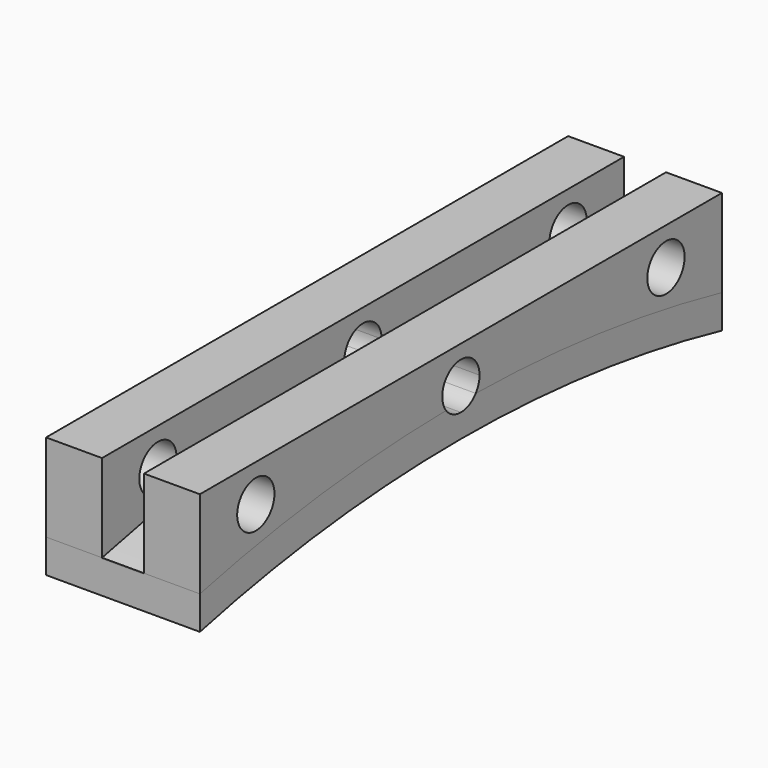
from build123d import *
from build123d import SkipClean  # not in build123d's __all__

# Parameters (mm, degrees)
F0_R     = 5
F1_DEPTH = 33
F2_W     = 9
F2_H     = 19
F3_DEPTH = 140
F5_DEPTH = 33


with BuildPart() as f1:
    # F0 (on Right) → F1 (new body)
    with BuildSketch(Plane.YZ):
        with BuildLine():
            ThreePointArc((0, 8), (35.2278299076, 5.9935116916), (70, 0))
            Line((70, 0), (70, 7.1810302798))
            ThreePointArc((70, 7.1810302798), (37.1952808389, 12.8120154562), (3.9811421818, 14.975019516))
            ThreePointArc((3.9811421818, 14.975019516), (2.2220595829, 13.5208872296), (0, 13))
            Line((0, 13), (0, 8))
        make_face()
        with BuildLine():
            ThreePointArc((3.9811421818, 14.975019516), (37.1952808389, 12.8120154562), (70, 7.1810302798))
            Line((70, 7.1810302798), (70, 26))
            Line((70, 26), (0, 26))
            Line((0, 26), (0, 23))
            ThreePointArc((0, 23), (3.5355339059, 21.5355339059), (5, 18))
            ThreePointArc((5, 18), (4.7384444129, 16.4040223856), (3.9811421818, 14.975019516))
        make_face()
        with Locations((55, 18)):
            Circle(F0_R, mode=Mode.SUBTRACT)
        with BuildLine():
            Line((-70, 26), (-70, 7.1810302798))
            ThreePointArc((-70, 7.1810302798), (-37.1952808389, 12.8120154562), (-3.9811421818, 14.975019516))
            ThreePointArc((-3.9811421818, 14.975019516), (-4.4791127704, 20.2220595829), (0, 23))
            Line((0, 23), (0, 26))
            Line((0, 26), (-70, 26))
        make_face()
        with Locations((-55, 18)):
            Circle(F0_R, mode=Mode.SUBTRACT)
        with BuildLine():
            Line((-70, 7.1810302798), (-70, 0))
            ThreePointArc((-70, 0), (-35.2278299076, 5.9935116916), (0, 8))
            Line((0, 8), (0, 13))
            ThreePointArc((0, 13), (-2.2220595829, 13.5208872296), (-3.9811421818, 14.975019516))
            ThreePointArc((-3.9811421818, 14.975019516), (-37.1952808389, 12.8120154562), (-70, 7.1810302798))
        make_face()
    extrude(amount=F1_DEPTH)

    # F2 (on face) → F3 (cut)
    with BuildSketch(Plane.XZ.offset(70)):
        with Locations((16.5, 16.5)):
            Rectangle(F2_W, F2_H)
    extrude(amount=-F3_DEPTH, mode=Mode.SUBTRACT)

    # F4 (on face) → F5 (join)
    with BuildSketch(Plane.YZ.offset(33)):
        with BuildLine():
            Line((70, 0), (70, 7.1810302798))
            ThreePointArc((70, 7.1810302798), (37.1952808389, 12.8120154562), (3.9811421818, 14.975019516))
            ThreePointArc((3.9811421818, 14.975019516), (0, 13), (-3.9811421818, 14.975019516))
            ThreePointArc((-3.9811421818, 14.975019516), (-37.1952808389, 12.8120154562), (-70, 7.1810302798))
            Line((-70, 7.1810302798), (-70, 0))
            ThreePointArc((-70, 0), (0, 8), (70, 0))
        make_face()
    with SkipClean():  # cleaning this boolean's faces spoils the solid; the shape is the same uncleaned
        extrude(amount=-F5_DEPTH)


solid = f1.part
